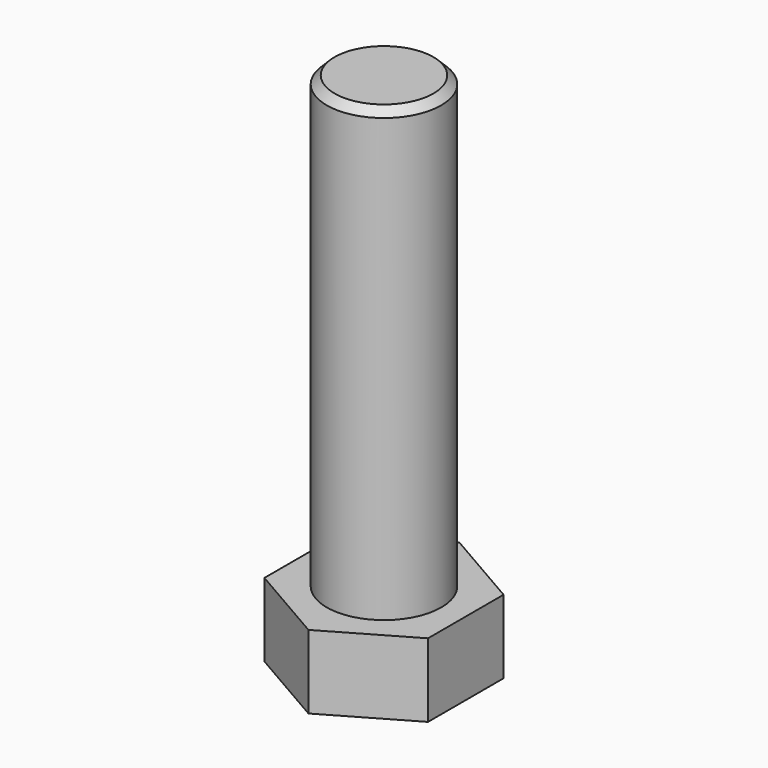
from build123d import *

# Parameters (mm, degrees)
F2_DEPTH = 7.14375
F0_R     = 5.55625
F3_DEPTH = 50.8
F5_SIZE  = 0.762


# Not quite as in the source:
# - a length typed as a fraction of an inch, garbled in the dataset ("3 / 203.2 mm" for 3/8 in), is restored


with BuildPart() as f2:
    # F1 (on Top) → F2 (new body)
    with BuildSketch(Plane.XY):
        Polygon((7.9375, 4.5827177617), (0, 9.1654355234), (-7.9375, 4.5827177617), (-7.9375, -4.5827177617), (0, -9.1654355234), (7.9375, -4.5827177617), align=None)
    extrude(amount=F2_DEPTH)

    # F0 (on Top) → F3 (join)
    with BuildSketch(Plane.XY):
        Circle(F0_R)
    extrude(amount=F3_DEPTH)

    # F5
    f5_edges = [f2.edges().sort_by_distance(p)[0] for p in [
        (-5.55625, 0, 50.8),
    ]]
    chamfer(f5_edges, length=F5_SIZE)


solid = f2.part
